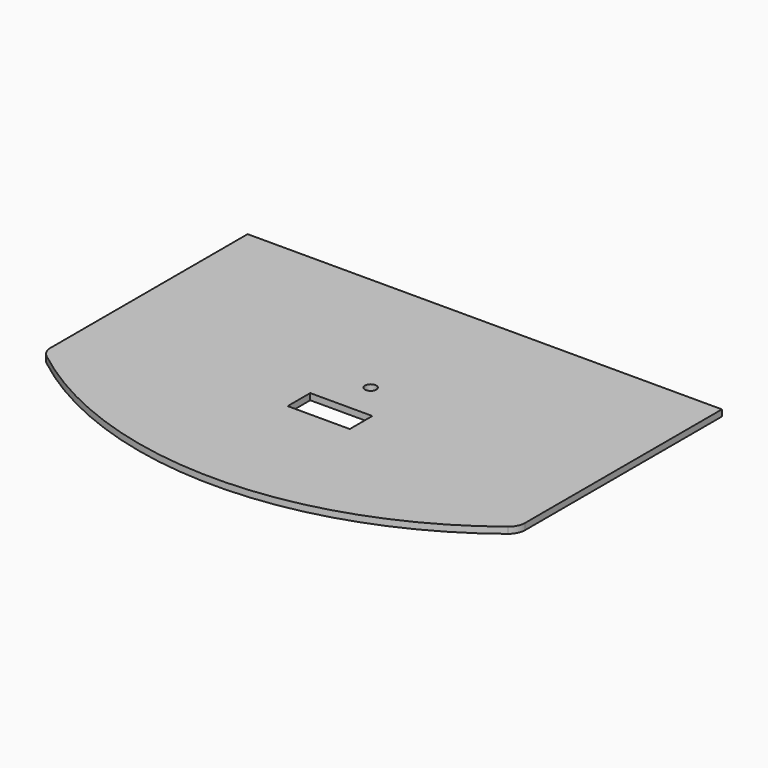
from build123d import *

# Parameters (mm, degrees)
F1_DEPTH = 28.575


# Not quite as in the source:
# - a feature names something its author has since deleted; it is built from what else it names


with BuildPart() as f1:
    # F0 (on Top) → F1 (new body)
    with BuildSketch(Plane.XY):
        with BuildLine():
            ThreePointArc((-1037.5478672986, -524.8695620945), (-548.7202955818, -790.5538516378), (0, -882.4590952158))
            ThreePointArc((0, -882.4590952158), (548.7202955818, -790.5538516378), (1037.5478672986, -524.8695620945))
            ThreePointArc((1037.5478672986, -524.8695620945), (1059.0976915237, -498.2343056164), (1066.8, -464.8500839552))
            Line((1066.8, -464.8500839552), (1066.8, -44.2590952158))
            Line((1066.8, -44.2590952158), (1066.8, 641.5409047842))
            Line((1066.8, 641.5409047842), (-1066.8, 641.5409047842))
            Line((-1066.8, 641.5409047842), (-1066.8, -44.2590952158))
            Line((-1066.8, -44.2590952158), (-1066.8, -464.8500839552))
            ThreePointArc((-1066.8, -464.8500839552), (-1059.0976915237, -498.2343056164), (-1037.5478672986, -524.8695620945))
        make_face()
        Polygon((-139.7, -165.1), (0, -165.1), (139.7, -165.1), (139.7, -292.1), (0, -292.1), (-139.7, -292.1), align=None, mode=Mode.SUBTRACT)
        with BuildLine():
            ThreePointArc((0, -25.4), (-17.9605122421, 17.9605122421), (25.4, 0))
            ThreePointArc((25.4, 0), (17.9605122421, -17.9605122421), (0, -25.4))
        make_face(mode=Mode.SUBTRACT)
    extrude(amount=F1_DEPTH)


solid = f1.part
